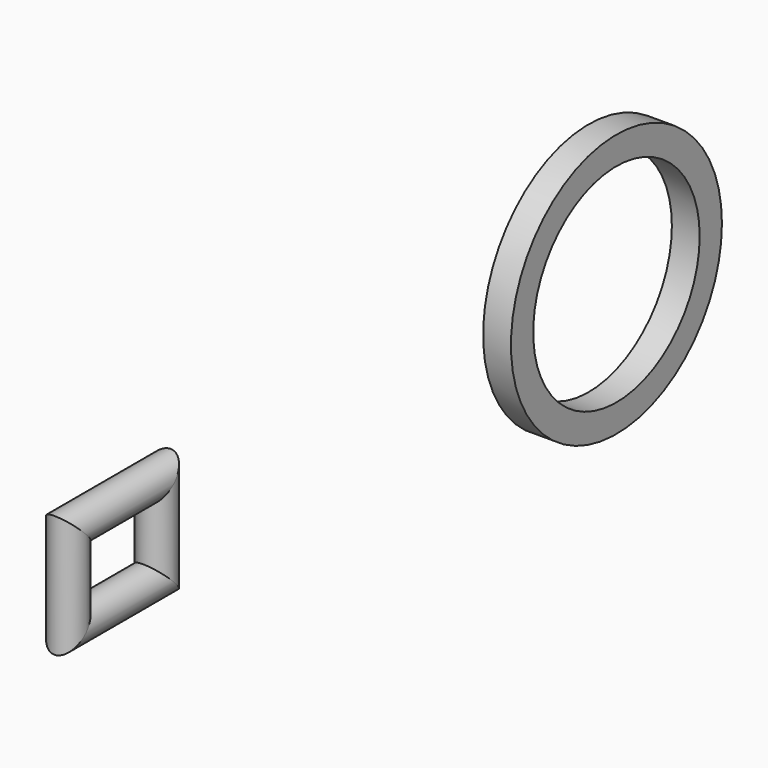
from build123d import *

# Parameters (mm, degrees)
F5_R = 12.5
F8_W = 20
F8_H = 20


# Not quite as in the source:
# - the program builds the solid bodies; features that only make, move or delete a surface that nothing else refers to are left out


with BuildPart() as f6:
    # F6: sweep along a path in F4
    with BuildLine(Plane.YZ) as f6_path:
        Line((-237.0753139257, 37.8463640809), (-237.0753139257, -24.9928794801))
        Line((-237.0753139257, -24.9928794801), (-157.574146986, -24.9928794801))
        Line((-157.574146986, -24.9928794801), (-157.574146986, 37.8463640809))
        Line((-157.574146986, 37.8463640809), (-237.0753139257, 37.8463640809))
    # F5 (on Top) → F6 (sweep)
    with BuildSketch(Plane.XY):
        with Locations((0, -237.0753139257)):
            Circle(F5_R)
    sweep(path=f6_path.line, transition=Transition.RIGHT)


with BuildPart() as f9:
    # F9: sweep along a path in F7
    with BuildLine(Plane.YZ) as f9_path:
        CenterArc((243.0302351713, 0), 50, 0, 360)
    # F8 (on Top) → F9 (sweep)
    with BuildSketch(Plane.XY):
        with Locations((0, 158.2333147526)):
            Rectangle(F8_W, F8_H)
    sweep(path=f9_path.line)


solid = Compound([f6.part, f9.part])
